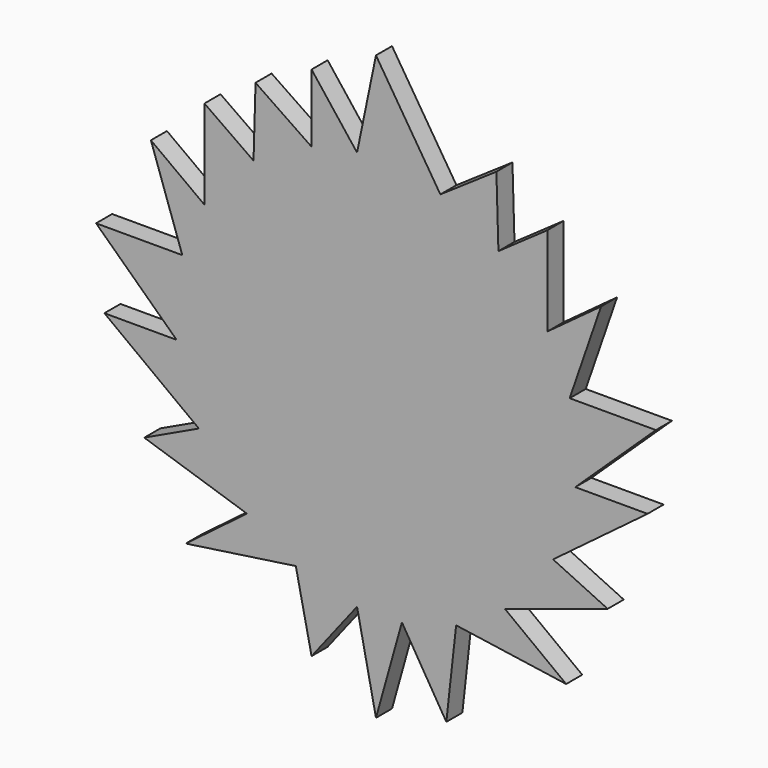
from build123d import *

# Parameters (mm, degrees)
F1_DEPTH = 6.35
F2_DEPTH = 6.35
F3_DEPTH = 6.35
F4_DEPTH = 6.35
F5_DEPTH = 6.35


# Not quite as in the source:
# - a feature names something its author has since deleted; it is built from what else it names


with BuildPart() as f1:
    # F0 (on Front) → F1 (new body)
    with BuildSketch(Plane.XZ):
        with BuildLine():
            ThreePointArc((63.0566746496, -7.490379305), (63.3890717721, -3.751743578), (63.5, 0))
            ThreePointArc((63.5, 0), (62.9393473013, 8.4195345051), (61.2672894084, 16.6903939003))
            ThreePointArc((61.2672894084, 16.6903939003), (58.3327446269, 25.0906537239), (54.2527974979, 32.9982418266))
            ThreePointArc((54.2527974979, 32.9982418266), (47.291532101, 42.3764202304), (38.730412603, 50.3210208521))
            ThreePointArc((38.730412603, 50.3210208521), (29.9555685969, 55.9903019284), (20.3699341201, 60.1441250991))
            ThreePointArc((20.3699341201, 60.1441250991), (7.3544916147, 63.0726680353), (-5.9855682874, 63.2172679912))
            ThreePointArc((-5.9855682874, 63.2172679912), (-13.2670335267, 62.09859758), (-20.3699341201, 60.1441250991))
            ThreePointArc((-20.3699341201, 60.1441250991), (-29.9555685969, 55.9903019284), (-38.730412603, 50.3210208521))
            ThreePointArc((-38.730412603, 50.3210208521), (-47.291532101, 42.3764202304), (-54.2527974979, 32.9982418266))
            ThreePointArc((-54.2527974979, 32.9982418266), (-58.3327446269, 25.0906537239), (-61.2672894084, 16.6903939003))
            ThreePointArc((-61.2672894084, 16.6903939003), (-63.3268462658, 4.6862076377), (-63.0566746496, -7.490379305))
            ThreePointArc((-63.0566746496, -7.490379305), (-60.5844983842, -19.0202143924), (-56.023116606, -29.8941533708))
            ThreePointArc((-56.023116606, -29.8941533708), (-49.318773707, -39.9988569841), (-40.8158107072, -48.6448311366))
            ThreePointArc((-40.8158107072, -48.6448311366), (-33.4288158961, -53.9885568226), (-25.3527004473, -58.2193316694))
            ThreePointArc((-25.3527004473, -58.2193316694), (-15.8671551858, -61.4856356095), (-5.9855682874, -63.2172679912))
            ThreePointArc((-5.9855682874, -63.2172679912), (1.1186954333, -63.4901450662), (8.2089360928, -62.9671610304))
            ThreePointArc((8.2089360928, -62.9671610304), (16.9479005402, -61.1965576424), (25.3527004473, -58.2193316694))
            ThreePointArc((25.3527004473, -58.2193316694), (33.4288158961, -53.9885568226), (40.8158107072, -48.6448311366))
            ThreePointArc((40.8158107072, -48.6448311366), (49.318773707, -39.9988569841), (56.023116606, -29.8941533708))
            ThreePointArc((56.023116606, -29.8941533708), (60.5844983842, -19.0202143924), (63.0566746496, -7.490379305))
        make_face()
        with BuildLine():
            ThreePointArc((61.2672894084, 16.6903939003), (62.9393473013, 8.4195345051), (63.5, 0))
            ThreePointArc((63.5, 0), (63.3890717721, -3.751743578), (63.0566746496, -7.490379305))
            Line((63.0566746496, -7.490379305), (88.5324627161, 16.6903939003))
            Line((88.5324627161, 16.6903939003), (61.2672894084, 16.6903939003))
        make_face()
        with BuildLine():
            ThreePointArc((54.2527974979, 32.9982418266), (58.3327446269, 25.0906537239), (61.2672894084, 16.6903939003))
            Line((61.2672894084, 16.6903939003), (71.193754673, 45.4481393099))
            Line((71.193754673, 45.4481393099), (54.2527974979, 32.9982418266))
        make_face()
        with BuildLine():
            Line((85.9054028988, -7.490379305), (63.0566746496, -7.490379305))
            ThreePointArc((63.0566746496, -7.490379305), (60.5844983842, -19.0202143924), (56.023116606, -29.8941533708))
            Line((56.023116606, -29.8941533708), (85.9054028988, -7.490379305))
        make_face()
        with BuildLine():
            ThreePointArc((38.730412603, 50.3210208521), (47.291532101, 42.3764202304), (54.2527974979, 32.9982418266))
            Line((54.2527974979, 32.9982418266), (54.2527974979, 61.2032547377))
            Line((54.2527974979, 61.2032547377), (38.730412603, 50.3210208521))
        make_face()
        with BuildLine():
            ThreePointArc((20.3699341201, 60.1441250991), (29.9555685969, 55.9903019284), (38.730412603, 50.3210208521))
            Line((38.730412603, 50.3210208521), (38.0926132202, 72.2317844629))
            Line((38.0926132202, 72.2317844629), (20.3699341201, 60.1441250991))
        make_face()
        with BuildLine():
            Line((60.1600408554, -63.261911273), (40.8158107072, -48.6448311366))
            ThreePointArc((40.8158107072, -48.6448311366), (33.4288158961, -53.9885568226), (25.3527004473, -58.2193316694))
            Line((25.3527004473, -58.2193316694), (60.1600408554, -63.261911273))
        make_face()
        with BuildLine():
            ThreePointArc((-20.3699341201, 60.1441250991), (-13.2670335267, 62.09859758), (-5.9855682874, 63.2172679912))
            Line((-5.9855682874, 63.2172679912), (-20.3699341201, 81.6848352551))
            Line((-20.3699341201, 81.6848352551), (-20.3699341201, 60.1441250991))
        make_face()
        with BuildLine():
            ThreePointArc((-38.730412603, 50.3210208521), (-29.9555685969, 55.9903019284), (-20.3699341201, 60.1441250991))
            Line((-20.3699341201, 60.1441250991), (-38.0926132202, 72.2317844629))
            Line((-38.0926132202, 72.2317844629), (-38.730412603, 50.3210208521))
        make_face()
        with BuildLine():
            ThreePointArc((-54.2527974979, 32.9982418266), (-47.291532101, 42.3764202304), (-38.730412603, 50.3210208521))
            Line((-38.730412603, 50.3210208521), (-54.2527974979, 61.2032547377))
            Line((-54.2527974979, 61.2032547377), (-54.2527974979, 32.9982418266))
        make_face()
        with BuildLine():
            Line((-60.1600408554, -63.261911273), (-25.3527004473, -58.2193316694))
            ThreePointArc((-25.3527004473, -58.2193316694), (-33.4288158961, -53.9885568226), (-40.8158107072, -48.6448311366))
            Line((-40.8158107072, -48.6448311366), (-60.1600408554, -63.261911273))
        make_face()
        with BuildLine():
            ThreePointArc((-61.2672894084, 16.6903939003), (-58.3327446269, 25.0906537239), (-54.2527974979, 32.9982418266))
            Line((-54.2527974979, 32.9982418266), (-71.193754673, 45.4481393099))
            Line((-71.193754673, 45.4481393099), (-61.2672894084, 16.6903939003))
        make_face()
        with BuildLine():
            ThreePointArc((-63.0566746496, -7.490379305), (-63.3268462658, 4.6862076377), (-61.2672894084, 16.6903939003))
            Line((-61.2672894084, 16.6903939003), (-88.5324627161, 16.6903939003))
            Line((-88.5324627161, 16.6903939003), (-63.0566746496, -7.490379305))
        make_face()
        with BuildLine():
            Line((-85.9054028988, -7.490379305), (-56.023116606, -29.8941533708))
            ThreePointArc((-56.023116606, -29.8941533708), (-60.5844983842, -19.0202143924), (-63.0566746496, -7.490379305))
            Line((-63.0566746496, -7.490379305), (-85.9054028988, -7.490379305))
        make_face()
    extrude(amount=F1_DEPTH)

    # F0 (on Front) → F2 (join)
    with BuildSketch(Plane.XZ):
        with BuildLine():
            Line((-73.2954144478, -38.053765893), (-40.8158107072, -48.6448311366))
            ThreePointArc((-40.8158107072, -48.6448311366), (-49.318773707, -39.9988569841), (-56.023116606, -29.8941533708))
            Line((-56.023116606, -29.8941533708), (-73.2954144478, -38.053765893))
        make_face()
        with BuildLine():
            Line((73.2954144478, -38.053765893), (56.023116606, -29.8941533708))
            ThreePointArc((56.023116606, -29.8941533708), (49.318773707, -39.9988569841), (40.8158107072, -48.6448311366))
            Line((40.8158107072, -48.6448311366), (73.2954144478, -38.053765893))
        make_face()
    extrude(amount=F2_DEPTH)

    # F0 (on Front) → F3 (join)
    with BuildSketch(Plane.XZ):
        with BuildLine():
            Line((0, -92.2421216965), (8.2089360928, -62.9671610304))
            ThreePointArc((8.2089360928, -62.9671610304), (1.1186954333, -63.4901450662), (-5.9855682874, -63.2172679912))
            Line((-5.9855682874, -63.2172679912), (0, -92.2421216965))
        make_face()
        with BuildLine():
            ThreePointArc((-5.9855682874, 63.2172679912), (7.3544916147, 63.0726680353), (20.3699341201, 60.1441250991))
            Line((20.3699341201, 60.1441250991), (0, 92.2421216965))
            Line((0, 92.2421216965), (-5.9855682874, 63.2172679912))
        make_face()
    extrude(amount=F3_DEPTH)

    # F0 (on Front) → F4 (join)
    with BuildSketch(Plane.XZ):
        with BuildLine():
            Line((-20.3699341201, -81.6848352551), (-5.9855682874, -63.2172679912))
            ThreePointArc((-5.9855682874, -63.2172679912), (-15.8671551858, -61.4856356095), (-25.3527004473, -58.2193316694))
            Line((-25.3527004473, -58.2193316694), (-20.3699341201, -81.6848352551))
        make_face()
        with BuildLine():
            Line((60.1600408554, -63.261911273), (40.8158107072, -48.6448311366))
            ThreePointArc((40.8158107072, -48.6448311366), (33.4288158961, -53.9885568226), (25.3527004473, -58.2193316694))
            Line((25.3527004473, -58.2193316694), (60.1600408554, -63.261911273))
        make_face()
    extrude(amount=F4_DEPTH)

    # F0 (on Front) → F5 (join)
    with BuildSketch(Plane.XZ):
        with BuildLine():
            Line((22.25664258, -86.1358046532), (25.3527004473, -58.2193316694))
            ThreePointArc((25.3527004473, -58.2193316694), (16.9479005402, -61.1965576424), (8.2089360928, -62.9671610304))
            Line((8.2089360928, -62.9671610304), (22.25664258, -86.1358046532))
        make_face()
    extrude(amount=F5_DEPTH)


solid = f1.part
